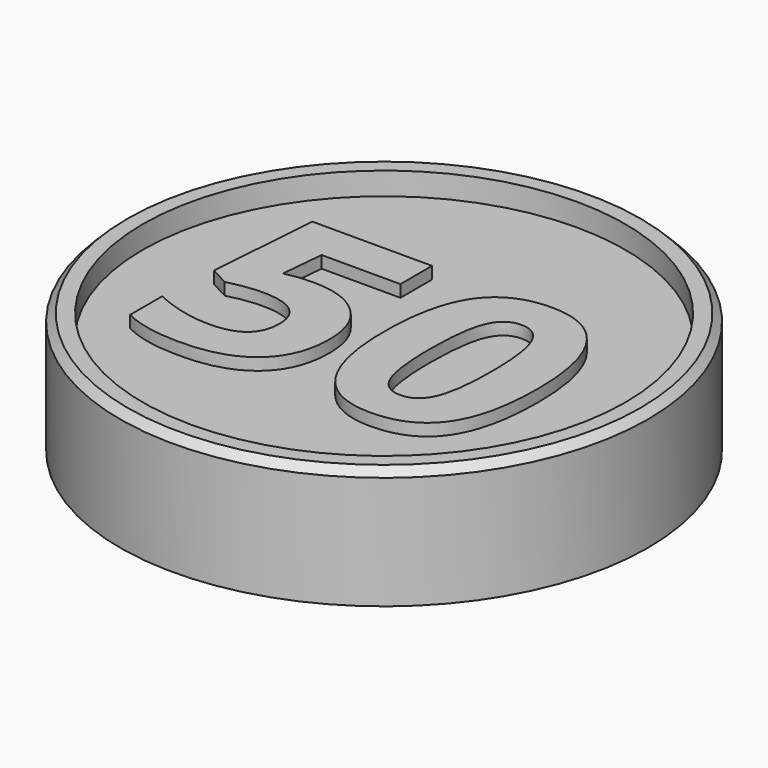
from build123d import *

# Parameters (mm, degrees)
F0_R         = 17.5
F1_DEPTH     = 8
F2_R         = 16
F3_DEPTH     = 1.5
F4_SIZE      = 0.5
F5_TEXT_SIZE = 20.4991325237
F6_DEPTH     = 0.8


# Not quite as in the source:
# - Text() gives the source's letters only with a copy of the font that has no kerning and outlines rounded to 1/6400 em; it was checked with that copy


with BuildPart() as f1:
    # F0 (on Top) → F1 (new body)
    with BuildSketch(Plane.XY):
        Circle(F0_R)
    extrude(amount=F1_DEPTH)

    # F2 (on face) → F3 (cut)
    with BuildSketch(Plane.XY.offset(8)):
        Circle(F2_R)
    extrude(amount=-F3_DEPTH, mode=Mode.SUBTRACT)

    # F4
    f4_edges = [f1.edges().sort_by_distance(p)[0] for p in [
        (-17.5, 0, 8),
    ]]
    chamfer(f4_edges, length=F4_SIZE)

    # F5 (on face) → F6 (join)
    with BuildSketch(Plane.XY.offset(6.5)):
        with Locations((-12, -7.8826142069)):
            Text('50', F5_TEXT_SIZE, font='Open Sans', font_style=FontStyle.BOLD, text_align=(TextAlign.LEFT, TextAlign.BOTTOM))
    extrude(amount=F6_DEPTH)


solid = f1.part
